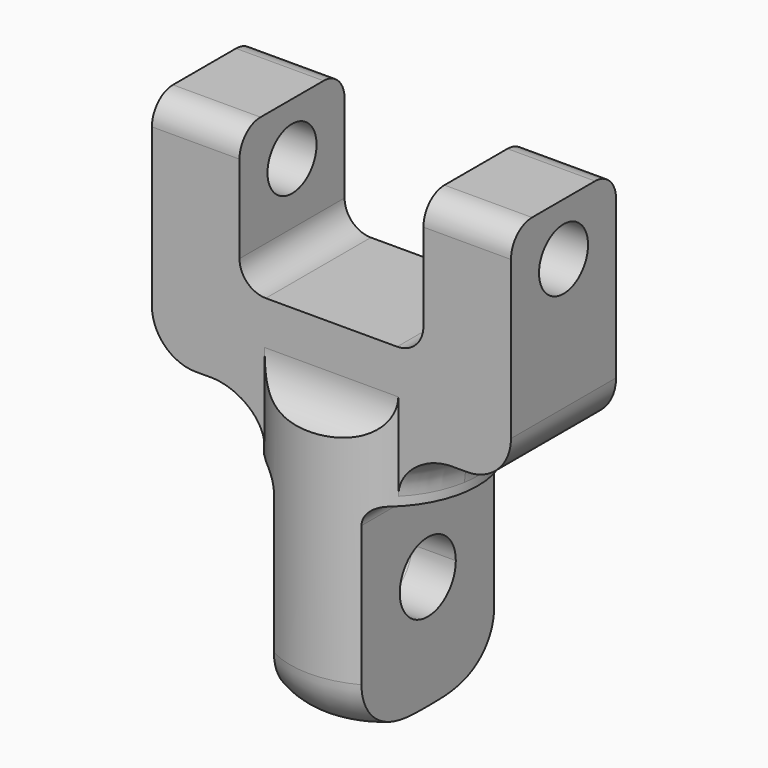
from build123d import *

# Parameters (mm, degrees)
F0_R          = 10.7
F1_DEPTH      = 30
F2_R          = 6
F3_W          = 41
F3_H          = 15
F4_DEPTH      = 10
F5_W          = 10
F5_H          = 16
F6_DEPTH      = 15
F8_DEPTH      = 20.501
F9_DEPTH      = 20.501
F10_W         = 10
F10_H         = 15
F11_DEPTH     = 16
F13_T4_DEPTH  = 40.2630272227
F13_S5_R      = 10.7
F13_T6_DEPTH  = 22
F13_T10_DEPTH = 40.2630272227
F13_S11_R     = 10.7
F13_T12_DEPTH = 22
F13_T13_DEPTH = 40
F14_D         = 7
F15_R         = 5
F16_W         = 6.2500013784
F16_H         = 36.9480545221
F16_W_2       = 6.8020046502
F16_H_2       = 40.0000055429
F17_DEPTH     = 24
F18_R         = 2
F19_R         = 3


# Not quite as in the source:
# - a fillet or chamfer that OpenCascade refuses, or shapes differently, is made with other operations: its cross-section is extruded or revolved along the edge and cut away or added
# - a feature names something its author has since deleted; it is built from what else it names


with BuildPart() as f1:
    # F0 (on Top) → F1 (new body)
    with BuildSketch(Plane.XY):
        Circle(F0_R)
    extrude(amount=-F1_DEPTH)

    # F2
    f2_edges = [f1.edges().sort_by_distance(p)[0] for p in [
        (-10.7, 0, -30),
    ]]
    fillet(f2_edges, radius=F2_R)

    # F3 (on face) → F4 (join)
    with BuildSketch(Plane.XY):
        Rectangle(F3_W, F3_H)
    extrude(amount=F4_DEPTH)

    # F5 (on face) → F6 (join)
    with BuildSketch(Plane(origin=(0, 7.5, 0), x_dir=(-1, 0, 0), z_dir=(0, 1, 0))):
        with Locations((15.5, 18)):
            Rectangle(F5_W, F5_H)
    extrude(amount=-F6_DEPTH)

    # F7 (on Right) → F8 (cut, through all)
    with BuildSketch(Plane.YZ):
        with BuildLine():
            ThreePointArc((0, -13), (-2.8284271247, -19.8284271247), (4, -17))
            ThreePointArc((4, -17), (2.8284271247, -14.1715728753), (0, -13))
        make_face()
    extrude(amount=-F8_DEPTH, mode=Mode.SUBTRACT)

    # F9 (cut, through all): a face of the model
    f9_faces = [f1.faces().sort_by_distance(p)[0] for p in [
        (0, 0, -17),
    ]]
    extrude(f9_faces, amount=-F9_DEPTH, mode=Mode.SUBTRACT)

    # F10 (on face) → F11 (join)
    with BuildSketch(Plane.XY.offset(10)):
        with Locations((15.5, 0)):
            Rectangle(F10_W, F10_H)
    extrude(amount=F11_DEPTH)

    # F13: fillet of radius 5 on 8 edges, made by hand


with BuildPart() as f13_tool2:
    # F13_s3 → F13_t4 (new body)
    with BuildSketch(Plane.YZ.offset(-20.1315136113)):
        with BuildLine():
            ThreePointArc((-12.5, 0), (-8.9644660941, 1.4644660941), (-7.5, 5))
            Line((-7.5, 5), (-7.5, 0))
            Line((-7.5, 0), (-12.5, 0))
        make_face()
    extrude(amount=F13_T4_DEPTH)

    # F13_s5 → F13_t6 (intersect, symmetric)
    with BuildSketch(Plane.XY.offset(2.5)):
        Circle(F13_S5_R)
    extrude(amount=F13_T6_DEPTH, both=True, mode=Mode.INTERSECT)


with BuildPart() as f1_1:
    add(f1.part)

    # F13_t1: union F13_tool2
    add(f13_tool2.part)


with BuildPart() as f13_tool8:
    # F13_s9 → F13_t10 (new body)
    with BuildSketch(Plane.YZ.offset(20.1315136113)):
        with BuildLine():
            ThreePointArc((7.5, 5), (8.9644660941, 1.4644660941), (12.5, 0))
            Line((12.5, 0), (7.5, 0))
            Line((7.5, 0), (7.5, 5))
        make_face()
    extrude(amount=-F13_T10_DEPTH)

    # F13_s11 → F13_t12 (intersect, symmetric)
    with BuildSketch(Plane.XY.offset(2.5)):
        Circle(F13_S11_R)
    extrude(amount=F13_T12_DEPTH, both=True, mode=Mode.INTERSECT)


with BuildPart() as f1_2:
    add(f1_1.part)

    # F13_t7: union F13_tool8
    add(f13_tool8.part)

    # F13_s14 → F13_t13 (cut)
    with BuildSketch(Plane.XZ.offset(-20)):
        with BuildLine():
            ThreePointArc((-15.5, 0), (-19.0355339059, 1.4644660941), (-20.5, 5))
            Line((-20.5, 5), (-20.5, 0))
            Line((-20.5, 0), (-15.5, 0))
        make_face()
        with BuildLine():
            ThreePointArc((15.5, 0), (19.0355339059, 1.4644660941), (20.5, 5))
            Line((20.5, 5), (20.5, 0))
            Line((20.5, 0), (15.5, 0))
        make_face()
    extrude(amount=F13_T13_DEPTH, mode=Mode.SUBTRACT)

    # F14 (through all)
    with Locations(Plane.YZ.offset(20.5)):
        with Locations((0, 20)):
            Hole(F14_D / 2)

    # F15
    f15_edges = [f1_2.edges().sort_by_distance(p)[0] for p in [
        (9.903211, 4.051716, 0),
        (-10.7, 0, 0),
        (9.903211, -4.051716, 0),
    ]]
    fillet(f15_edges, radius=F15_R)

    # F16 (on face) → F17 (cut)
    with BuildSketch(Plane(origin=(0, 0, -30), x_dir=(1, 0, 0), z_dir=(0, 0, -1))):
        with Locations((-8.1250006892, 1.5259755104)):
            Rectangle(F16_W, F16_H)
        with Locations((8.4010023251, 0)):
            Rectangle(F16_W_2, F16_H_2)
    extrude(amount=-F17_DEPTH, mode=Mode.SUBTRACT)

    # F18
    f18_edges = [f1_2.edges().sort_by_distance(p)[0] for p in [
        (-5, 0, -6),
        (5, 0, -6),
    ]]
    fillet(f18_edges, radius=F18_R)

    # F19
    f19_edges = [f1_2.edges().sort_by_distance(p)[0] for p in [
        (10.5, 0, 10),
        (-10.5, 0, 10),
        (15.5, -7.5, 26),
        (-15.5, -7.5, 26),
        (-15.5, 7.5, 26),
        (15.5, 7.5, 26),
    ]]
    fillet(f19_edges, radius=F19_R)


solid = f1_2.part
